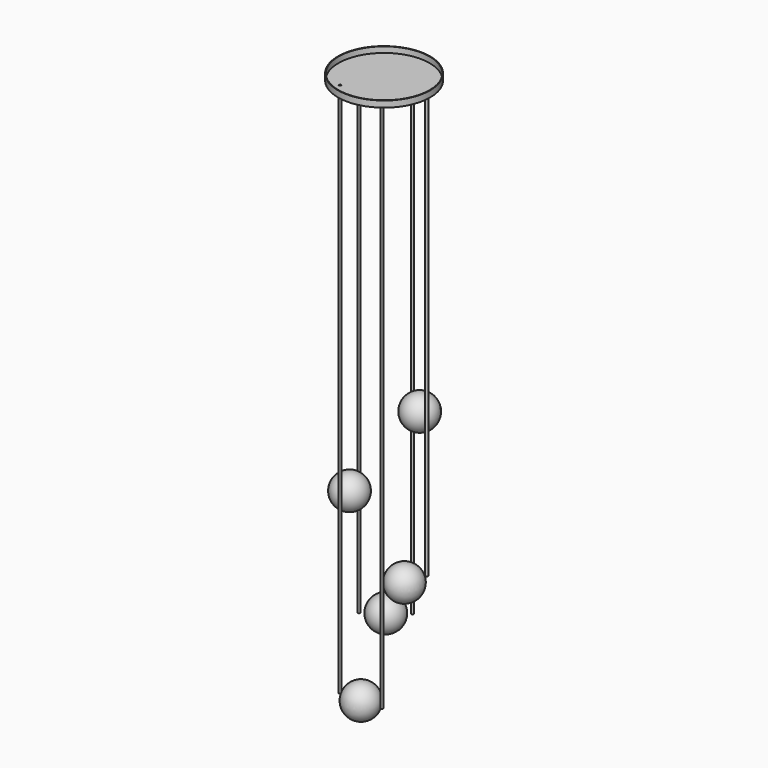
from build123d import *

# Parameters (mm, degrees)
F7_R      = 7.9375
F8_DEPTH  = 3238.5
F13_DEPTH = 2933.7
F14_DEPTH = 2603.5
F27_R     = 279.4
F27_R_2   = 7.9375
F28_DEPTH = 38.1
F29_R     = 276.225
F30_DEPTH = 34.925


with BuildPart() as f8:
    # F7 (on plane+point) → F8 (new body, through all)
    with BuildSketch(Plane.XY.offset(4203.7)):
        with Locations((7213.6, -174.8005038998)):
            Circle(F7_R)
    extrude(amount=-F8_DEPTH)


with BuildPart() as f8b:
    # F7 (on plane+point) → F8, piece 2 (new body, through all)
    with BuildSketch(Plane.XY.offset(4203.7)):
        with Locations((6959.6, -174.8005038998)):
            Circle(F7_R)
    extrude(amount=-F8_DEPTH)


with BuildPart() as f13:
    # F7 (on plane+point) → F13 (new body, through all)
    with BuildSketch(Plane.XY.offset(4203.7)):
        with Locations((6881.1096834288, 66.7678512391)):
            Circle(F7_R)
    extrude(amount=-F13_DEPTH)


with BuildPart() as f13b:
    # F7 (on plane+point) → F13, piece 2 (new body, through all)
    with BuildSketch(Plane.XY.offset(4203.7)):
        with Locations((7086.6, 216.0653053214)):
            Circle(F7_R)
    extrude(amount=-F13_DEPTH)


with BuildPart() as f14:
    # F7 (on plane+point) → F14 (new body, through all)
    with BuildSketch(Plane.XY.offset(4203.7)):
        with Locations((7292.0903165712, 66.7678512391)):
            Circle(F7_R)
    extrude(amount=-F14_DEPTH)


with BuildPart() as f16:
    # F15 (on plane+point) → F16 (revolve)
    with BuildSketch(Plane.XY.offset(965.2)):
        with BuildLine():
            ThreePointArc((6985, -174.8005038998), (7086.6, -276.4005038998), (7188.2, -174.8005038998))
            Line((7188.2, -174.8005038998), (6985, -174.8005038998))
        make_face()
    revolve(axis=Axis((7086.6, -174.8005038998, 965.2), (-1, 0, 0)))


with BuildPart() as f18:
    # F17 (on plane+point) → F18 (revolve)
    with BuildSketch(Plane.XY.offset(1981.2)):
        with BuildLine():
            ThreePointArc((6888.9587150859, 42.6110157252), (6823.7274996588, -85.4124529589), (6951.7509683429, -150.6436683859))
            Line((6951.7509683429, -150.6436683859), (6888.9587150859, 42.6110157252))
        make_face()
    revolve(axis=Axis((6920.3548417144, -54.0163263304, 1981.2), (-0.3090169944, 0.9510565163, 0)))


with BuildPart() as f20:
    # F19 (on plane+point) → F20 (revolve)
    with BuildSketch(Plane.XY.offset(1270)):
        with BuildLine():
            ThreePointArc((7066.0509683429, 201.1355599132), (6924.1358600815, 223.6127049088), (6901.6587150859, 81.6975966474))
            Line((6901.6587150859, 81.6975966474), (7066.0509683429, 201.1355599132))
        make_face()
    revolve(axis=Axis((6983.8548417144, 141.4165782803, 1270), (0.8090169944, 0.5877852523, 0)))


with BuildPart() as f22:
    # F21 (on plane+point) → F22 (revolve)
    with BuildSketch(Plane.XY.offset(2413)):
        with BuildLine():
            ThreePointArc((7271.5412849141, 81.6975966474), (7249.0641399185, 223.6127049088), (7107.1490316571, 201.1355599132))
            Line((7107.1490316571, 201.1355599132), (7271.5412849141, 81.6975966474))
        make_face()
    revolve(axis=Axis((7189.3451582856, 141.4165782803, 2413), (0.8090169944, -0.5877852523, 0)))


with BuildPart() as f24:
    # F23 (on plane+point) → F24 (revolve)
    with BuildSketch(Plane.XY.offset(1600.2)):
        with BuildLine():
            ThreePointArc((7221.4490316571, -150.6436683859), (7349.4725003412, -85.4124529588), (7284.2412849141, 42.6110157252))
            Line((7284.2412849141, 42.6110157252), (7221.4490316571, -150.6436683859))
        make_face()
    revolve(axis=Axis((7252.8451582856, -54.0163263304, 1600.2), (-0.3090169944, -0.9510565163, 0)))


with BuildPart() as f26:
    # F23 (on plane+point) → F26 (revolve)
    with BuildSketch(Plane.XY.offset(1600.2)):
        with BuildLine():
            ThreePointArc((7221.4490316571, -150.6436683859), (7349.4725003412, -85.4124529588), (7284.2412849141, 42.6110157252))
            Line((7284.2412849141, 42.6110157252), (7221.4490316571, -150.6436683859))
        make_face()
    revolve(axis=Axis((7252.8451582856, -54.0163263304, 1600.2), (-0.3090169944, -0.9510565163, 0)))


with BuildPart() as f28:
    # F27 (on face) → F28 (new body)
    with BuildSketch(Plane.XY.offset(4203.7)):
        with Locations((7086.6, 0)):
            Circle(F27_R)
        with Locations((6959.6, -174.8005038998)):
            Circle(F27_R_2, mode=Mode.SUBTRACT)
    extrude(amount=F28_DEPTH)

    # F29 (on face) → F30 (cut)
    with BuildSketch(Plane.XY.offset(4241.8)):
        with Locations((7086.6, 0)):
            Circle(F29_R)
    extrude(amount=-F30_DEPTH, mode=Mode.SUBTRACT)


solid = Compound([f8.part, f8b.part, f13.part, f13b.part, f14.part, f16.part, f18.part, f20.part, f22.part, f24.part, f26.part, f28.part])
